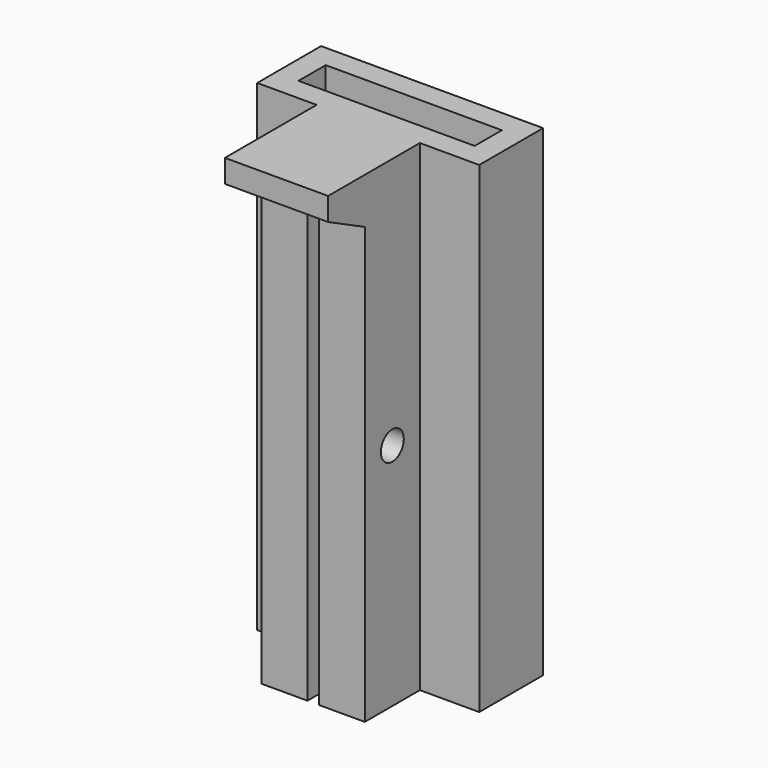
from build123d import *

# Parameters (mm, degrees)
F1_DEPTH = 53.34
F2_R     = 1.5875
F3_DEPTH = 25.4
F4_W     = 1.27
F4_H     = 5.08
F4_H_2   = 7.62
F5_DEPTH = 50.8
F7_DEPTH = 5.08


with BuildPart() as f1:
    # F0 (on Top) → F1 (new body)
    with BuildSketch(Plane.XY):
        Polygon((12.2936, 0), (6.5786, 0), (6.5786, -12.7), (18.0086, -12.7), (18.0086, 0), align=None)
        Polygon((0, 8.8392), (0, 0), (6.5786, 0), (12.2936, 0), (12.2936, 2.54), (2.54, 2.54), (2.54, 6.2992), (5.08, 6.2992), (12.2936, 6.2992), (12.2936, 8.8392), (5.08, 8.8392), align=None)
        Polygon((12.2936, 2.54), (12.2936, 0), (18.0086, 0), (24.5872, 0), (24.5872, 8.8392), (19.5072, 8.8392), (12.2936, 8.8392), (12.2936, 6.2992), (19.5072, 6.2992), (22.0472, 6.2992), (22.0472, 2.54), align=None)
    extrude(amount=F1_DEPTH)

    # F2 (on face) → F3 (cut)
    with BuildSketch(Plane.YZ.offset(18.0086)):
        Polygon((-7.62, 48.26), (-12.7, 50.8), (-12.7, 0), (-7.62, 0), align=None)
        with Locations((-3.81, 25.4)):
            Circle(F2_R)
    extrude(amount=-F3_DEPTH, mode=Mode.SUBTRACT)

    # F4 (on face) → F5 (cut)
    with BuildSketch(Plane(origin=(0, 0, 0), x_dir=(1, 0, 0), z_dir=(0, 0, -1))):
        with Locations((12.2936, 10.16)):
            Rectangle(F4_W, F4_H)
        with Locations((12.2936, 3.81)):
            Rectangle(F4_W, F4_H_2)
    extrude(amount=-F5_DEPTH, mode=Mode.SUBTRACT)

    # F6 (on face) → F7 (cut)
    with BuildSketch(Plane(origin=(0, 8.8392, 0), x_dir=(-1, 0, 0), z_dir=(0, 1, 0))):
        with BuildLine():
            ThreePointArc((-10.7061, 25.4), (-11.1710679849, 26.5225320151), (-12.2936, 26.9875))
            Line((-12.2936, 26.9875), (-12.2936, 25.4))
            Line((-12.2936, 25.4), (-10.7061, 25.4))
        make_face()
        with BuildLine():
            Line((-12.2936, 25.4), (-12.2936, 26.9875))
            ThreePointArc((-12.2936, 26.9875), (-13.4161320151, 26.5225320151), (-13.8811, 25.4))
            Line((-13.8811, 25.4), (-12.2936, 25.4))
        make_face()
        with BuildLine():
            Line((-10.7061, 25.4), (-12.2936, 25.4))
            Line((-12.2936, 25.4), (-12.2936, 23.8125))
            ThreePointArc((-12.2936, 23.8125), (-11.1710679849, 24.2774679849), (-10.7061, 25.4))
        make_face()
        with BuildLine():
            Line((-12.2936, 23.8125), (-12.2936, 25.4))
            Line((-12.2936, 25.4), (-13.8811, 25.4))
            ThreePointArc((-13.8811, 25.4), (-13.4161320151, 24.2774679849), (-12.2936, 23.8125))
        make_face()
    extrude(amount=-F7_DEPTH, mode=Mode.SUBTRACT)


solid = f1.part
